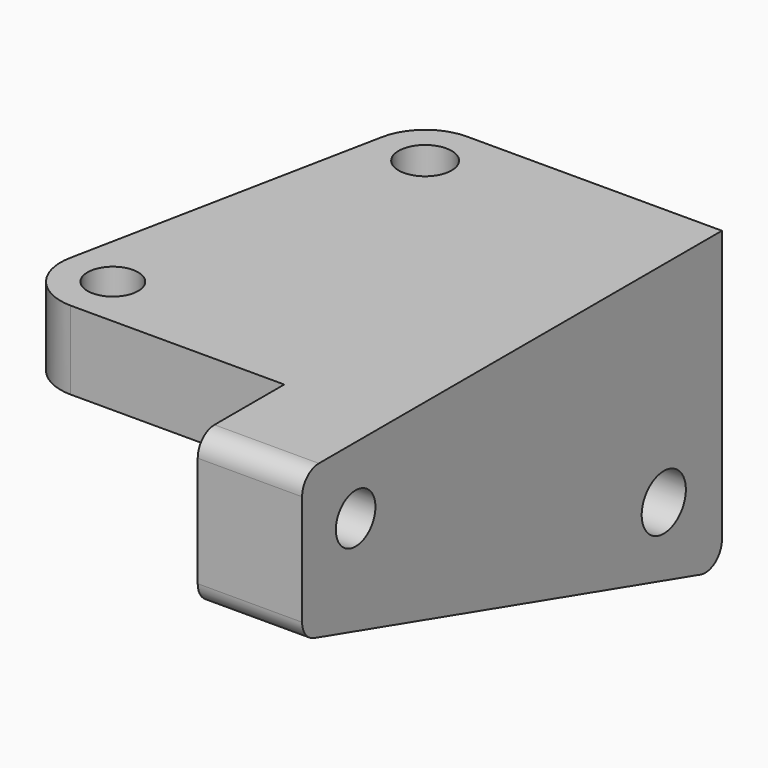
from build123d import *

# Parameters (mm, degrees)
F0_R     = 6.717517972
F0_R_2   = 6.020799142
F0_W     = 93.3380946517
F0_H     = 25.1572784036
F1_DEPTH = 25.4
F2_R     = 6.1623070593
F2_R_2   = 6.4550817185
F3_DEPTH = 19.05
F4_R     = 5.08


with BuildPart() as f1:
    # F0 (on Right) → F1 (new body)
    with BuildSketch(Plane.YZ):
        Polygon((-29.2035490274, 0), (-63.4982287884, 0), (-63.4982287884, -35.7638783753), (64.1345456243, -72.88698107), (64.1345456243, -25.1572784036), (-29.2035490274, -25.1572784036), align=None)
        with Locations((46.4568771422, -50.9666763246)):
            Circle(F0_R, mode=Mode.SUBTRACT)
        with Locations((-47.2347699106, -16.3184423)):
            Circle(F0_R_2, mode=Mode.SUBTRACT)
        with Locations((17.4654982984, -12.5786392018)):
            Rectangle(F0_W, F0_H)
    extrude(amount=F1_DEPTH)

    # F2 (on Top) → F3 (join)
    with BuildSketch(Plane.XY):
        with BuildLine():
            Line((-49.083184828, 53.9312161083), (-64.3051586518, -21.9885608041))
            ThreePointArc((-64.3051586518, -21.9885608041), (-61.737725203, -32.4590575274), (-52.0475044965, -37.1837415174))
            Line((-52.0475044965, -37.1837415174), (25.4, -37.1837415174))
            Line((25.4, -37.1837415174), (25.4, 64.1345456243))
            Line((25.4, 64.1345456243), (-36.6310108614, 64.1345456243))
            ThreePointArc((-36.6310108614, 64.1345456243), (-44.6803053911, 61.2579288283), (-49.083184828, 53.9312161083))
        make_face()
        with Locations((-51.8529846852, -24.4852312881)):
            Circle(F2_R, mode=Mode.SUBTRACT)
        with Locations((-36.6310108614, 51.4345456243)):
            Circle(F2_R_2, mode=Mode.SUBTRACT)
    extrude(amount=-F3_DEPTH)

    # F4
    f4_edges = [f1.edges().sort_by_distance(p)[0] for p in [
        (12.7, 64.134546, -72.886981),
        (12.7, -63.498229, -35.763878),
        (12.7, -63.498229, 0),
        (0, 13.475402, -19.05),
    ]]
    fillet(f4_edges, radius=F4_R)


solid = f1.part
